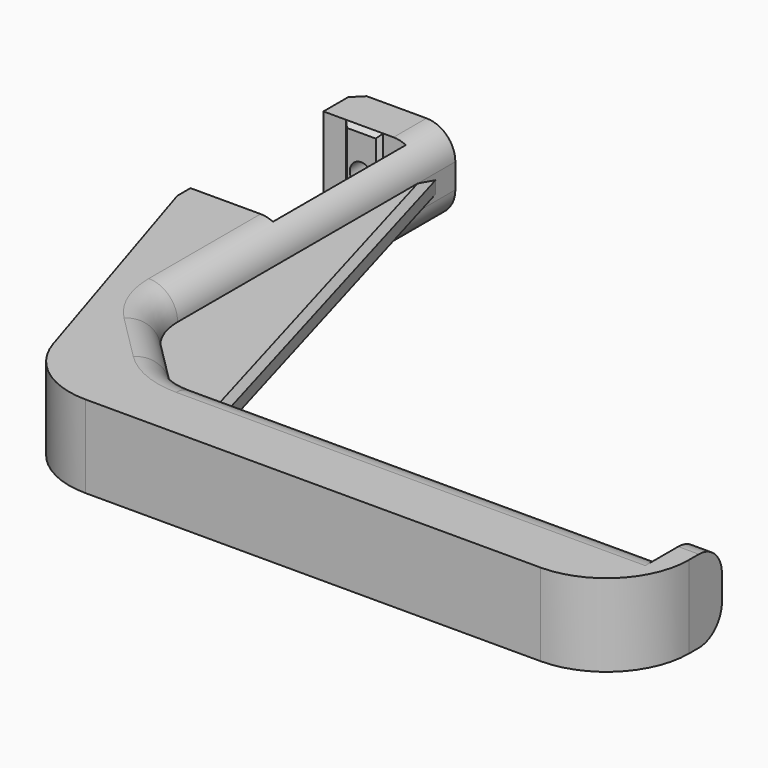
from build123d import *

# Parameters (mm, degrees)
F1_DEPTH      = 20
F2_W          = 9
F2_H          = 1
F3_DEPTH      = 20
F4_SIZE       = 0.99999
F6_DEPTH      = 20
F9_DEPTH      = 3
F10_SIZE      = 20
F11_DEPTH     = 6
F13_R         = 2.8
F14_DEPTH     = 130.4192752567
F15_R         = 6
F16_DEPTH     = 76.1192752567
F17_R         = 6
F18_DEPTH     = 6
F19_R         = 15
F20_T1_DEPTH  = 113.7867965644
F20_T3_DEPTH  = 40
F20_T5_DEPTH  = 15.8578643763
F20_T7_DEPTH  = 101.7050718211
F20_T10_ANGLE = 45
F20_T12_ANGLE = 45
F20_T14_ANGLE = 45
F20_T16_ANGLE = 45
F21_SIZE      = 1.5
F22_R         = 20
F23_SIZE      = 2.5


# Not quite as in the source:
# - a fillet or chamfer that OpenCascade refuses, or shapes differently, is made with other operations: its cross-section is extruded or revolved along the edge and cut away or added
# - a fillet or chamfer is up to 0.001 mm smaller than in the source, because OpenCascade refuses the exact size


with BuildPart() as f1:
    # F0 (on Top) → F1 (new body)
    with BuildSketch(Plane.XY):
        Polygon((24, 0), (0, 0), (0, -4), (20, -4), (20, -44.3), (0, -44.3), (0, -48.3), (24, -48.3), align=None)
    extrude(amount=F1_DEPTH)

    # F2 (on face) → F3 (join, through all)
    with BuildSketch(Plane.XY.offset(20)):
        with Locations((10, -4.5)):
            Rectangle(F2_W, F2_H)
        with Locations((10, -43.8)):
            Rectangle(F2_W, F2_H)
    extrude(amount=-F3_DEPTH)

    # F4 (size 1 in the source; OpenCascade refuses exactly that, so slightly less here)
    f4_edges = [f1.edges().sort_by_distance(p)[0] for p in [
        (5.5, -5, 10),
        (14.5, -5, 10),
        (10, -5, 20),
        (10, -5, 0),
        (14.5, -43.3, 10),
        (5.5, -43.3, 10),
        (10, -43.3, 20),
        (10, -43.3, 0),
    ]]
    chamfer(f4_edges, length=F4_SIZE)

    # F5 (on face) → F6 (join, through all)
    with BuildSketch(Plane.XY.offset(20)):
        Polygon((24, -48.3), (0, -48.3), (24, -124.4182752567), (169, -124.4182752567), (169, -94.4182752567), (164, -94.4182752567), (164, -104.4182752567), (24, -104.4182752567), align=None)
    extrude(amount=-F6_DEPTH)

    # F8 (on offset) → F9 (join, symmetric)
    with BuildSketch(Plane.XY.offset(10)):
        Polygon((54, -104.4182752567), (24, 0), (24, -104.4182752567), align=None)
    extrude(amount=F9_DEPTH, both=True)

    # F10
    f10_edges = [f1.edges().sort_by_distance(p)[0] for p in [
        (24, -104.418275, 16.5),
        (24, -104.418275, 3.5),
    ]]
    chamfer(f10_edges, length=F10_SIZE)

    # F11 (add): a face of the model
    f11_faces = [f1.faces().sort_by_distance(p)[0] for p in [
        (12, 0, 10),
    ]]
    extrude(f11_faces, amount=F11_DEPTH)

    # F13 (on face) → F14 (cut, through all)
    with BuildSketch(Plane(origin=(0, 6, 0), x_dir=(-1, 0, 0), z_dir=(0, 1, 0))):
        with Locations((-10, 10)):
            Circle(F13_R)
    extrude(amount=-F14_DEPTH, mode=Mode.SUBTRACT)

    # F15 (on offset) → F16 (cut, through all)
    with BuildSketch(Plane(origin=(0, -48.3, 0), x_dir=(-1, 0, 0), z_dir=(0, 1, 0))):
        with Locations((-10, 10)):
            Circle(F15_R)
    extrude(amount=-F16_DEPTH, mode=Mode.SUBTRACT)

    # F17 (on face) → F18 (cut)
    with BuildSketch(Plane(origin=(0, 6, 0), x_dir=(-1, 0, 0), z_dir=(0, 1, 0))):
        with Locations((-10, 10)):
            Circle(F17_R)
    extrude(amount=-F18_DEPTH, mode=Mode.SUBTRACT)

    # F19
    f19_edges = [f1.edges().sort_by_distance(p)[0] for p in [
        (44, -104.418275, 3.5),
        (24, -84.418275, 3.5),
        (24, -84.418275, 16.5),
        (44, -104.418275, 16.5),
    ]]
    fillet(f19_edges, radius=F19_R)

    # F20: fillet of radius 7 on 12 edges, made by hand

    # F20_s2 → F20_t1 (cut)
    with BuildSketch(Plane.YZ.offset(50.2132034356)):
        with BuildLine():
            ThreePointArc((-104.4182752567, 13), (-106.4685277884, 17.9497474683), (-111.4182752567, 20))
            Line((-111.4182752567, 20), (-104.4182752567, 20))
            Line((-104.4182752567, 20), (-104.4182752567, 13))
        make_face()
        with BuildLine():
            ThreePointArc((-111.4182752567, 0), (-106.4685277884, 2.0502525317), (-104.4182752567, 7))
            Line((-104.4182752567, 7), (-104.4182752567, 0))
            Line((-104.4182752567, 0), (-111.4182752567, 0))
        make_face()
    extrude(amount=F20_T1_DEPTH, mode=Mode.SUBTRACT)

    # F20_s4 → F20_t3 (cut)
    with BuildSketch(Plane.YZ.offset(146.5)):
        with BuildLine():
            ThreePointArc((-101.4182752567, 0), (-96.4685277884, 2.0502525317), (-94.4182752567, 7))
            Line((-94.4182752567, 7), (-94.4182752567, 0))
            Line((-94.4182752567, 0), (-101.4182752567, 0))
        make_face()
        with BuildLine():
            ThreePointArc((-94.4182752567, 13), (-96.4685277884, 17.9497474683), (-101.4182752567, 20))
            Line((-101.4182752567, 20), (-94.4182752567, 20))
            Line((-94.4182752567, 20), (-94.4182752567, 13))
        make_face()
    extrude(amount=F20_T3_DEPTH, mode=Mode.SUBTRACT)

    # F20_s6 → F20_t5 (cut)
    with BuildSketch(Plane(origin=(69.8157393462, -69.8157393462, 0), x_dir=(0, 0, 1), z_dir=(-0.7071067812, 0.7071067812, 0))):
        with BuildLine():
            ThreePointArc((0, -49.7221721416), (2.0502525317, -44.7724246733), (7, -42.7221721416))
            Line((7, -42.7221721416), (0, -42.7221721416))
            Line((0, -42.7221721416), (0, -49.7221721416))
        make_face()
        with BuildLine():
            ThreePointArc((20, -49.7221721416), (17.9497474683, -44.7724246733), (13, -42.7221721416))
            Line((13, -42.7221721416), (20, -42.7221721416))
            Line((20, -42.7221721416), (20, -49.7221721416))
        make_face()
    extrude(amount=F20_T5_DEPTH, mode=Mode.SUBTRACT)

    # F20_s8 → F20_t7 (cut)
    with BuildSketch(Plane.XZ.offset(-23.5)):
        with BuildLine():
            ThreePointArc((17, 0), (21.9497474683, 2.0502525317), (24, 7))
            Line((24, 7), (24, 0))
            Line((24, 0), (17, 0))
        make_face()
        with BuildLine():
            ThreePointArc((24, 13), (21.9497474683, 17.9497474683), (17, 20))
            Line((17, 20), (24, 20))
            Line((24, 20), (24, 13))
        make_face()
    extrude(amount=F20_T7_DEPTH, mode=Mode.SUBTRACT)

    # F20_s9 → F20_t10 (revolve, cut)
    with BuildSketch(Plane.YZ.offset(50.2132034356)):
        with BuildLine():
            ThreePointArc((-111.4182752567, 0), (-106.4685277884, 2.0502525317), (-104.4182752567, 7))
            Line((-104.4182752567, 7), (-104.4182752567, 0))
            Line((-104.4182752567, 0), (-111.4182752567, 0))
        make_face()
    revolve(axis=Axis((50.2132034356, -89.4182752567, 0), (0, 0, -1)), revolution_arc=F20_T10_ANGLE, mode=Mode.SUBTRACT)

    # F20_s11 → F20_t12 (revolve, cut)
    with BuildSketch(Plane(origin=(58.6025359106, -58.6025359106, 0), x_dir=(0, 0, 1), z_dir=(0.7071067812, -0.7071067812, 0))):
        with BuildLine():
            ThreePointArc((0, 49.7221721416), (2.0502525317, 44.7724246733), (7, 42.7221721416))
            Line((7, 42.7221721416), (0, 42.7221721416))
            Line((0, 42.7221721416), (0, 49.7221721416))
        make_face()
    revolve(axis=Axis((39, -78.2050718211, 0), (0, 0, -1)), revolution_arc=F20_T12_ANGLE, mode=Mode.SUBTRACT)

    # F20_s13 → F20_t14 (revolve, cut)
    with BuildSketch(Plane.YZ.offset(50.2132034356)):
        with BuildLine():
            ThreePointArc((-111.4182752567, 20), (-106.4685277884, 17.9497474683), (-104.4182752567, 13))
            Line((-104.4182752567, 13), (-104.4182752567, 20))
            Line((-104.4182752567, 20), (-111.4182752567, 20))
        make_face()
    revolve(axis=Axis((50.2132034356, -89.4182752567, 20), (0, 0, -1)), revolution_arc=F20_T14_ANGLE, mode=Mode.SUBTRACT)

    # F20_s15 → F20_t16 (revolve, cut)
    with BuildSketch(Plane.XZ.offset(78.2050718211)):
        with BuildLine():
            ThreePointArc((17, 20), (21.9497474683, 17.9497474683), (24, 13))
            Line((24, 13), (24, 20))
            Line((24, 20), (17, 20))
        make_face()
    revolve(axis=Axis((39, -78.2050718211, 20), (0, 0, 1)), revolution_arc=F20_T16_ANGLE, mode=Mode.SUBTRACT)

    # F21
    f21_edges = [f1.edges().sort_by_distance(p)[0] for p in [
        (39, -52.209138, 13),
        (39, -52.209138, 7),
    ]]
    chamfer(f21_edges, length=F21_SIZE)

    # F22
    f22_edges = [f1.edges().sort_by_distance(p)[0] for p in [
        (24, -124.418275, 10),
        (169, -124.418275, 10),
    ]]
    fillet(f22_edges, radius=F22_R)

    # F23
    f23_edges = [f1.edges().sort_by_distance(p)[0] for p in [
        (0, 6, 10),
    ]]
    chamfer(f23_edges, length=F23_SIZE)


solid = f1.part
